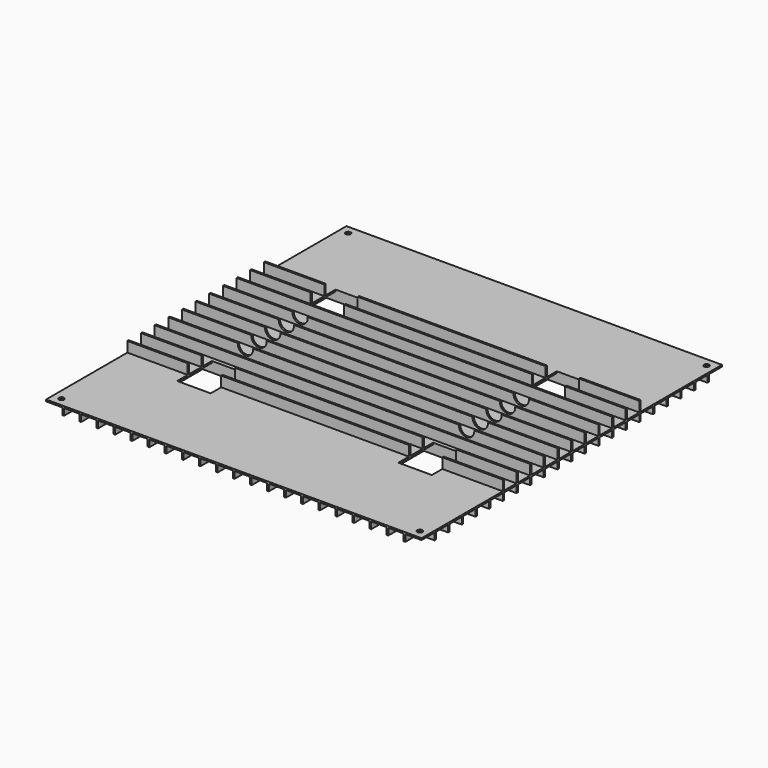
from build123d import *

# Parameters (mm, degrees)
F0_W      = 220
F0_H      = 220
F0_R      = 1.5
F1_DEPTH  = 1
F3_W      = 220
F3_H      = 1
F3_W_2    = 9.0000080466
F3_W_3    = 140
F3_W_4    = 31
F3_W_5    = 8.9999919534
F2_W      = 32.4
F2_H      = 27.4
F4_DEPTH  = 5
F5_DEPTH  = 6
F6_W      = 1
F6_H      = 220
F7_DEPTH  = 5
F2_W_2    = 5.4
F2_H_2    = 25.4
F2_W_3    = 19.6
F8_DEPTH  = 25
F9_DEPTH  = 25
F10_R     = 4.5
F11_DEPTH = 25


# Not quite as in the source:
# - a feature names something its author has since deleted; it is built from what else it names


with BuildPart() as f1:
    # F0 (on Top) → F1 (new body)
    with BuildSketch(Plane.XY):
        with Locations((8.0466e-06, 0.2085125446)):
            Rectangle(F0_W, F0_H)
        with Locations((-104.9999919534, -104.7914874554)):
            Circle(F0_R, mode=Mode.SUBTRACT)
        with Locations((105.0000080466, -104.7914874554)):
            Circle(F0_R, mode=Mode.SUBTRACT)
        with Locations((-104.9999919534, 105.2085125446)):
            Circle(F0_R, mode=Mode.SUBTRACT)
        with Locations((105.0000080466, 105.2085125446)):
            Circle(F0_R, mode=Mode.SUBTRACT)
    extrude(amount=-F1_DEPTH)

    # F3 (on Top) + F2 (on face) → F4 (join)
    with BuildSketch(Plane.XY):
        with Locations((5.96e-07, -79.7914874554)):
            Rectangle(F3_W, F3_H)
        with Locations((5.96e-07, -69.7914874554)):
            Rectangle(F3_W, F3_H)
        with Locations((5.96e-07, -59.7914874554)):
            Rectangle(F3_W, F3_H)
        with Locations((5.96e-07, -9.7914874554)):
            Rectangle(F3_W, F3_H)
        with Locations((5.96e-07, 0.2085125446)):
            Rectangle(F3_W, F3_H)
        with Locations((5.96e-07, 10.2085125446)):
            Rectangle(F3_W, F3_H)
        with Locations((5.96e-07, 60.2085125446)):
            Rectangle(F3_W, F3_H)
        with Locations((5.96e-07, 70.2085125446)):
            Rectangle(F3_W, F3_H)
        with Locations((5.96e-07, 80.2085125446)):
            Rectangle(F3_W, F3_H)
        with Locations((5.96e-07, 100.2085125446)):
            Rectangle(F3_W, F3_H)
        with Locations((5.96e-07, 90.2085125446)):
            Rectangle(F3_W, F3_H)
        with Locations((-105.4999953806, 50.2085125446)):
            Rectangle(F3_W_2, F3_H)
        with Locations((8.6427e-06, 50.2085125446)):
            Rectangle(F3_W_3, F3_H)
        with Locations((8.6427e-06, 40.2085125446)):
            Rectangle(F3_W_3, F3_H)
        with Locations((-105.4999953806, 40.2085125446)):
            Rectangle(F3_W_2, F3_H)
        with Locations((-105.4999953806, 30.2085125446)):
            Rectangle(F3_W_2, F3_H)
        with Locations((8.6427e-06, 30.2085125446)):
            Rectangle(F3_W_3, F3_H)
        with Locations((5.96e-07, 20.2085125446)):
            Rectangle(F3_W, F3_H)
        with Locations((85.5000086427, 50.2085125446)):
            Rectangle(F3_W_4, F3_H)
        with Locations((105.5000046194, 50.2085125446)):
            Rectangle(F3_W_5, F3_H)
        with Locations((85.5000086427, 40.2085125446)):
            Rectangle(F3_W_4, F3_H)
        with Locations((105.5000046194, 40.2085125446)):
            Rectangle(F3_W_5, F3_H)
        with Locations((85.5000086427, 30.2085125446)):
            Rectangle(F3_W_4, F3_H)
        with Locations((105.5000046194, 30.2085125446)):
            Rectangle(F3_W_5, F3_H)
        with Locations((-85.4999913573, 30.2085125446)):
            Rectangle(F3_W_4, F3_H)
        with Locations((-85.4999913573, 40.2085125446)):
            Rectangle(F3_W_4, F3_H)
        with Locations((-85.4999913573, 50.2085125446)):
            Rectangle(F3_W_4, F3_H)
        with Locations((-105.4999953806, -29.7914874554)):
            Rectangle(F3_W_2, F3_H)
        with Locations((-85.4999913573, -29.7914874554)):
            Rectangle(F3_W_4, F3_H)
        with Locations((-105.4999953806, -39.7914874554)):
            Rectangle(F3_W_2, F3_H)
        with Locations((-85.4999913573, -39.7914874554)):
            Rectangle(F3_W_4, F3_H)
        with Locations((5.96e-07, -19.7914874554)):
            Rectangle(F3_W, F3_H)
        with Locations((-105.4999953806, -49.7914874554)):
            Rectangle(F3_W_2, F3_H)
        with Locations((-85.4999913573, -49.7914874554)):
            Rectangle(F3_W_4, F3_H)
        with Locations((8.6427e-06, -49.7914874554)):
            Rectangle(F3_W_3, F3_H)
        with Locations((8.6427e-06, -39.7914874554)):
            Rectangle(F3_W_3, F3_H)
        with Locations((8.6427e-06, -29.7914874554)):
            Rectangle(F3_W_3, F3_H)
        with Locations((105.5000046194, -49.7914874554)):
            Rectangle(F3_W_5, F3_H)
        with Locations((105.5000046194, -39.7914874554)):
            Rectangle(F3_W_5, F3_H)
        with Locations((105.5000046194, -29.7914874554)):
            Rectangle(F3_W_5, F3_H)
        with Locations((85.5000086427, -29.7914874554)):
            Rectangle(F3_W_4, F3_H)
        with Locations((85.5000086427, -39.7914874554)):
            Rectangle(F3_W_4, F3_H)
        with Locations((85.5000086427, -49.7914874554)):
            Rectangle(F3_W_4, F3_H)
        with Locations((5.96e-07, -89.7914874554)):
            Rectangle(F3_W, F3_H)
        with Locations((5.96e-07, -99.7914874554)):
            Rectangle(F3_W, F3_H)
    with BuildSketch(Plane(origin=(0, 0, -1), x_dir=(1, 0, 0), z_dir=(0, 0, -1))):
        with Locations((64.8000080466, -45.2999696016)):
            Rectangle(F2_W, F2_H)
        Polygon((49.6000080466, -57.9999696016), (49.6000080466, -32.5999696016), (55.0000080466, -32.5999696016), (74.6000080466, -32.5999696016), (80.0000080466, -32.5999696016), (80.0000080466, -57.9999696016), (74.6000080466, -57.9999696016), (55.0000080466, -57.9999696016), align=None, mode=Mode.SUBTRACT)
        with Locations((64.8000080466, 45.2999696016)):
            Rectangle(F2_W, F2_H)
        Polygon((55.0000080466, 57.9999696016), (74.6000080466, 57.9999696016), (80.0000080466, 57.9999696016), (80.0000080466, 32.5999696016), (74.6000080466, 32.5999696016), (55.0000080466, 32.5999696016), (49.6000080466, 32.5999696016), (49.6000080466, 57.9999696016), align=None, mode=Mode.SUBTRACT)
        with Locations((-64.8000080466, 45.2999696016)):
            Rectangle(F2_W, F2_H)
        Polygon((-74.6000080466, 57.9999696016), (-55.0000080466, 57.9999696016), (-49.6000080466, 57.9999696016), (-49.6000080466, 32.5999696016), (-55.0000080466, 32.5999696016), (-74.6000080466, 32.5999696016), (-80.0000080466, 32.5999696016), (-80.0000080466, 57.9999696016), align=None, mode=Mode.SUBTRACT)
        with Locations((-64.8000080466, -45.2999696016)):
            Rectangle(F2_W, F2_H)
        Polygon((-49.6000080466, -32.5999696016), (-49.6000080466, -57.9999696016), (-55.0000080466, -57.9999696016), (-74.6000080466, -57.9999696016), (-80.0000080466, -57.9999696016), (-80.0000080466, -32.5999696016), (-74.6000080466, -32.5999696016), (-55.0000080466, -32.5999696016), align=None, mode=Mode.SUBTRACT)
    extrude(amount=-F4_DEPTH, dir=(0, 0, 1))

    # F3 (on Top) → F5 (join)
    with BuildSketch(Plane.XY):
        with Locations((-105.4999953806, 50.2085125446)):
            Rectangle(F3_W_2, F3_H)
        with Locations((-85.4999913573, 50.2085125446)):
            Rectangle(F3_W_4, F3_H)
        with Locations((8.6427e-06, 50.2085125446)):
            Rectangle(F3_W_3, F3_H)
        with Locations((85.5000086427, 50.2085125446)):
            Rectangle(F3_W_4, F3_H)
        with Locations((105.5000046194, 50.2085125446)):
            Rectangle(F3_W_5, F3_H)
        with Locations((-105.4999953806, 40.2085125446)):
            Rectangle(F3_W_2, F3_H)
        with Locations((-85.4999913573, 40.2085125446)):
            Rectangle(F3_W_4, F3_H)
        with Locations((8.6427e-06, 40.2085125446)):
            Rectangle(F3_W_3, F3_H)
        with Locations((85.5000086427, 40.2085125446)):
            Rectangle(F3_W_4, F3_H)
        with Locations((105.5000046194, 40.2085125446)):
            Rectangle(F3_W_5, F3_H)
        with Locations((-105.4999953806, 30.2085125446)):
            Rectangle(F3_W_2, F3_H)
        with Locations((-85.4999913573, 30.2085125446)):
            Rectangle(F3_W_4, F3_H)
        with Locations((8.6427e-06, 30.2085125446)):
            Rectangle(F3_W_3, F3_H)
        with Locations((85.5000086427, 30.2085125446)):
            Rectangle(F3_W_4, F3_H)
        with Locations((105.5000046194, 30.2085125446)):
            Rectangle(F3_W_5, F3_H)
        with Locations((5.96e-07, 20.2085125446)):
            Rectangle(F3_W, F3_H)
        with Locations((5.96e-07, 10.2085125446)):
            Rectangle(F3_W, F3_H)
        with Locations((5.96e-07, 0.2085125446)):
            Rectangle(F3_W, F3_H)
        with Locations((5.96e-07, -9.7914874554)):
            Rectangle(F3_W, F3_H)
        with Locations((5.96e-07, -19.7914874554)):
            Rectangle(F3_W, F3_H)
        with Locations((-105.4999953806, -29.7914874554)):
            Rectangle(F3_W_2, F3_H)
        with Locations((-85.4999913573, -29.7914874554)):
            Rectangle(F3_W_4, F3_H)
        with Locations((8.6427e-06, -29.7914874554)):
            Rectangle(F3_W_3, F3_H)
        with Locations((85.5000086427, -29.7914874554)):
            Rectangle(F3_W_4, F3_H)
        with Locations((105.5000046194, -29.7914874554)):
            Rectangle(F3_W_5, F3_H)
        with Locations((-105.4999953806, -39.7914874554)):
            Rectangle(F3_W_2, F3_H)
        with Locations((-85.4999913573, -39.7914874554)):
            Rectangle(F3_W_4, F3_H)
        with Locations((8.6427e-06, -39.7914874554)):
            Rectangle(F3_W_3, F3_H)
        with Locations((85.5000086427, -39.7914874554)):
            Rectangle(F3_W_4, F3_H)
        with Locations((105.5000046194, -39.7914874554)):
            Rectangle(F3_W_5, F3_H)
        with Locations((-105.4999953806, -49.7914874554)):
            Rectangle(F3_W_2, F3_H)
        with Locations((-85.4999913573, -49.7914874554)):
            Rectangle(F3_W_4, F3_H)
        with Locations((8.6427e-06, -49.7914874554)):
            Rectangle(F3_W_3, F3_H)
        with Locations((85.5000086427, -49.7914874554)):
            Rectangle(F3_W_4, F3_H)
        with Locations((105.5000046194, -49.7914874554)):
            Rectangle(F3_W_5, F3_H)
    extrude(amount=F5_DEPTH)

    # F6 (on Top) → F7 (join)
    with BuildSketch(Plane.XY):
        with Locations((80.0000080466, 0.2085125446)):
            Rectangle(F6_W, F6_H)
        with Locations((70.0000080466, 0.2085125446)):
            Rectangle(F6_W, F6_H)
        with Locations((60.0000080466, 0.2085125446)):
            Rectangle(F6_W, F6_H)
        with Locations((-9.9999919534, 0.2085125446)):
            Rectangle(F6_W, F6_H)
        with Locations((8.0466e-06, 0.2085125446)):
            Rectangle(F6_W, F6_H)
        with Locations((10.0000080466, 0.2085125446)):
            Rectangle(F6_W, F6_H)
        with Locations((-79.9999919534, 0.2085125446)):
            Rectangle(F6_W, F6_H)
        with Locations((-69.9999919534, 0.2085125446)):
            Rectangle(F6_W, F6_H)
        with Locations((-59.9999919534, 0.2085125446)):
            Rectangle(F6_W, F6_H)
        with Locations((-99.9999919534, 0.2085125446)):
            Rectangle(F6_W, F6_H)
        with Locations((-89.9999919534, 0.2085125446)):
            Rectangle(F6_W, F6_H)
        with Locations((-49.9999919534, 0.2085125446)):
            Rectangle(F6_W, F6_H)
        with Locations((-39.9999919534, 0.2085125446)):
            Rectangle(F6_W, F6_H)
        with Locations((-29.9999919534, 0.2085125446)):
            Rectangle(F6_W, F6_H)
        with Locations((-19.9999919534, 0.2085125446)):
            Rectangle(F6_W, F6_H)
        with Locations((20.0000080466, 0.2085125446)):
            Rectangle(F6_W, F6_H)
        with Locations((30.0000080466, 0.2085125446)):
            Rectangle(F6_W, F6_H)
        with Locations((40.0000080466, 0.2085125446)):
            Rectangle(F6_W, F6_H)
        with Locations((50.0000080466, 0.2085125446)):
            Rectangle(F6_W, F6_H)
        with Locations((90.0000080466, 0.2085125446)):
            Rectangle(F6_W, F6_H)
        with Locations((100.0000080466, 0.2085125446)):
            Rectangle(F6_W, F6_H)
    extrude(amount=-F7_DEPTH)

    # F2 (on face) → F8 (cut)
    with BuildSketch(Plane(origin=(0, 0, -1), x_dir=(1, 0, 0), z_dir=(0, 0, -1))):
        with Locations((77.3000080466, -45.2999696016)):
            Rectangle(F2_W_2, F2_H_2)
        with Locations((52.3000080466, -45.2999696016)):
            Rectangle(F2_W_2, F2_H_2)
        with Locations((64.8000080466, -45.2999696016)):
            Rectangle(F2_W_3, F2_H_2)
        with Locations((-52.3000080466, -45.2999696016)):
            Rectangle(F2_W_2, F2_H_2)
        with Locations((-64.8000080466, -45.2999696016)):
            Rectangle(F2_W_3, F2_H_2)
        with Locations((-77.3000080466, -45.2999696016)):
            Rectangle(F2_W_2, F2_H_2)
        with Locations((-52.3000080466, 45.2999696016)):
            Rectangle(F2_W_2, F2_H_2)
        with Locations((-64.8000080466, 45.2999696016)):
            Rectangle(F2_W_3, F2_H_2)
        with Locations((-77.3000080466, 45.2999696016)):
            Rectangle(F2_W_2, F2_H_2)
        with Locations((52.3000080466, 45.2999696016)):
            Rectangle(F2_W_2, F2_H_2)
        with Locations((64.8000080466, 45.2999696016)):
            Rectangle(F2_W_3, F2_H_2)
        with Locations((77.3000080466, 45.2999696016)):
            Rectangle(F2_W_2, F2_H_2)
    extrude(amount=F8_DEPTH, mode=Mode.SUBTRACT)

    # F2 (on face) → F9 (cut)
    with BuildSketch(Plane(origin=(0, 0, -1), x_dir=(1, 0, 0), z_dir=(0, 0, -1))):
        with Locations((64.8000080466, -45.2999696016)):
            Rectangle(F2_W_3, F2_H_2)
        with Locations((-64.8000080466, -45.2999696016)):
            Rectangle(F2_W_3, F2_H_2)
        with Locations((-64.8000080466, 45.2999696016)):
            Rectangle(F2_W_3, F2_H_2)
        with Locations((64.8000080466, 45.2999696016)):
            Rectangle(F2_W_3, F2_H_2)
    extrude(amount=-F9_DEPTH, mode=Mode.SUBTRACT)

    # F10 (on Front) → F11 (cut, symmetric)
    with BuildSketch(Plane.XZ):
        with Locations((64.7997068938, 5.5402468815)):
            Circle(F10_R)
        with Locations((-64.8002931062, 5.5402468815)):
            Circle(F10_R)
    extrude(amount=F11_DEPTH, both=True, mode=Mode.SUBTRACT)


solid = f1.part
